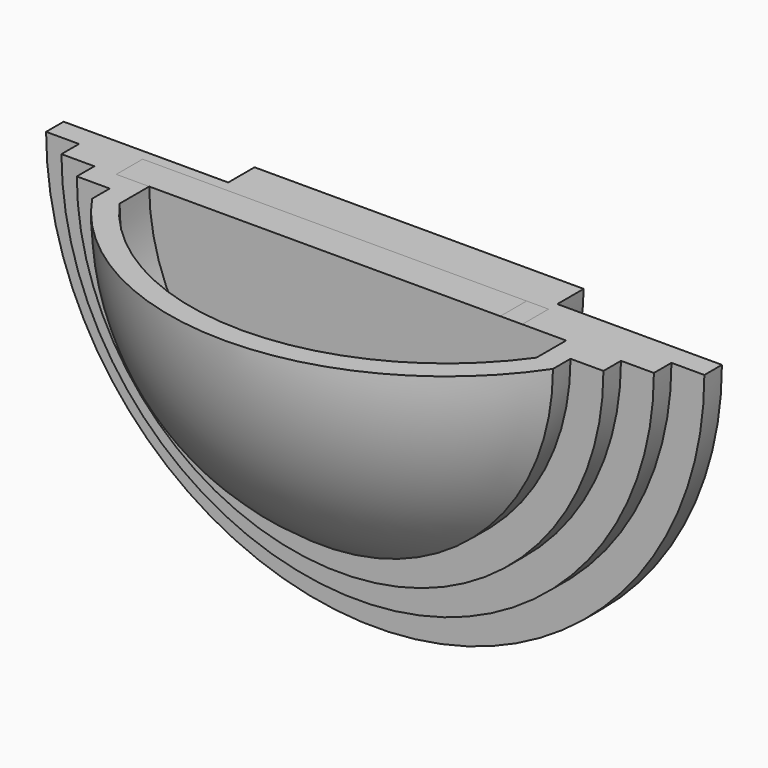
from build123d import *

# Parameters (mm, degrees)
F1_DEPTH      = 3
F2_DEPTH      = 2
F4_DEPTH      = 2
F5_DEPTH      = 4
F7_DEPTH      = 2
F9_ANGLE      = 180
F10_T         = 2
F10_T4_ANGLE  = 180.000000001
F10_T6_ANGLE  = 180.000000001
F10_T8_ANGLE  = 180.000000001
F10_T10_ANGLE = 180.000000001
F11_DEPTH     = 3
F12_DEPTH     = 1
F13_DEPTH     = 3


# Not quite as in the source:
# - a shell that OpenCascade refuses in one call is made with other operations: the cavity is built on its own and cut out


with BuildPart() as f1:
    # F0 (on Front) → F1 (new body)
    with BuildSketch(Plane.XZ):
        with BuildLine():
            Line((15, 0), (-15, 0))
            ThreePointArc((-15, 0), (0, -15), (15, 0))
        make_face()
    extrude(amount=-F1_DEPTH)

    # F0 (on Front) → F2 (join)
    with BuildSketch(Plane.XZ):
        with BuildLine():
            ThreePointArc((15, 0), (0, -15), (-15, 0))
            Line((-15, 0), (-30, 0))
            ThreePointArc((-30, 0), (0, -30), (30, 0))
            Line((30, 0), (15, 0))
        make_face()
        with BuildLine():
            Line((15, 0), (-15, 0))
            ThreePointArc((-15, 0), (0, -15), (15, 0))
        make_face()
    extrude(amount=F2_DEPTH)

    # F3 (on face) → F4 (join)
    with BuildSketch(Plane.XZ.offset(2)):
        with BuildLine():
            ThreePointArc((-27, 0), (0, -27), (27, 0))
            Line((27, 0), (24, 0))
            ThreePointArc((24, 0), (0, -24), (-24, 0))
            Line((-24, 0), (-27, 0))
        make_face()
    extrude(amount=F4_DEPTH)

    # F5 (add): a face of the model
    f5_faces = [f1.faces().sort_by_distance(p)[0] for p in [
        (0, -2, -10.1859163579),
    ]]
    extrude(f5_faces, amount=F5_DEPTH)

    # F6 (on face) → F7 (join)
    with BuildSketch(Plane.XZ.offset(6)):
        with BuildLine():
            ThreePointArc((-21, 0), (0, -21), (21, 0))
            Line((21, 0), (-21, 0))
        make_face()
    extrude(amount=F7_DEPTH)

    # F8 (on face) → F9 (revolve)
    with BuildSketch(Plane.XY):
        with BuildLine():
            Line((0, -8), (-21, -8))
            ThreePointArc((-21, -8), (-11.8972036761, -16.2165961892), (0, -19.1881107091))
            Line((0, -19.1881107091), (0, -8))
        make_face()
    revolve(axis=Axis((0, 0.2930196971, 0), (0, -1, 0)), revolution_arc=F9_ANGLE)

    # F10: shell of thickness 2, made by hand


with BuildPart() as f10_core1:
    # F10_t2: copy of F1
    add(f1.part)

    # the walls: a layer under each face that stays
    f10_faces = [f10_core1.faces().sort_by_distance(p)[0] for p in [
        (0, -1, -30),
        (-20, 0, -15),
        (-25.7142857143, -2, -15),
        (0, -3, -27),
        (-23.1428571429, -4, -13.5),
        (0, -5, -24),
        (-20.5714285714, -6, -12),
        (0, -7, -21),
        (0, 1.5, -15),
        (0, 3, -7.5),
        (0, -16.2165961892, -11.8972036761),
    ]]
    thicken(f10_faces, amount=-F10_T, mode=Mode.SUBTRACT)

    # F10_s3 → F10_t4 (revolve, cut)
    with BuildSketch(Plane.XY):
        Polygon((-15.02, 0.02), (-15, -2), (-13, -2), (-13, 0), align=None)
    revolve(axis=Axis((0, 0, 0), (0, -1, 0)), revolution_arc=F10_T4_ANGLE, mode=Mode.SUBTRACT)

    # F10_s5 → F10_t6 (revolve, cut)
    with BuildSketch(Plane.XY):
        Polygon((-27.02, -2.02), (-27, 0), (-25, 0), (-25, -2), align=None)
    revolve(axis=Axis((0, -2, 0), (0, -1, 0)), revolution_arc=F10_T6_ANGLE, mode=Mode.SUBTRACT)

    # F10_s7 → F10_t8 (revolve, cut)
    with BuildSketch(Plane.XY):
        Polygon((24.02, -4.02), (24, -2), (22, -2), (22, -4), align=None)
    revolve(axis=Axis((0, -4, 0), (0, 1, 0)), revolution_arc=F10_T8_ANGLE, mode=Mode.SUBTRACT)

    # F10_s9 → F10_t10 (revolve, cut)
    with BuildSketch(Plane.XY):
        Polygon((-21.02, -6.02), (-21, -4), (-19, -4), (-19, -6), align=None)
    revolve(axis=Axis((0, -6, 0), (0, -1, 0)), revolution_arc=F10_T10_ANGLE, mode=Mode.SUBTRACT)


with BuildPart() as f1_1:
    add(f1.part)

    # what is left inside the walls is the cavity
    f10_cavity = [f10_core1.part.solids().sort_by_distance(p)[0] for p in [
        (0, -12.621798, -13.821356),
    ]]
    add(f10_cavity, mode=Mode.SUBTRACT)

    # F11 (add, through all): a face of the model
    f11_faces = [f1_1.faces().sort_by_distance(p)[0] for p in [
        (0, 1, -5.5173713605),
    ]]
    extrude(f11_faces, amount=F11_DEPTH)

    # F12 (cut): a face of the model
    f12_faces = [f1_1.faces().sort_by_distance(p)[0] for p in [
        (0, -2, -9.3370899946),
    ]]
    extrude(f12_faces, amount=-F12_DEPTH, mode=Mode.SUBTRACT)

    # F13 (add): a face of the model
    f13_faces = [f1_1.faces().sort_by_distance(p)[0] for p in [
        (0, -1, -9.3370899946),
    ]]
    extrude(f13_faces, amount=F13_DEPTH)


solid = f1_1.part
